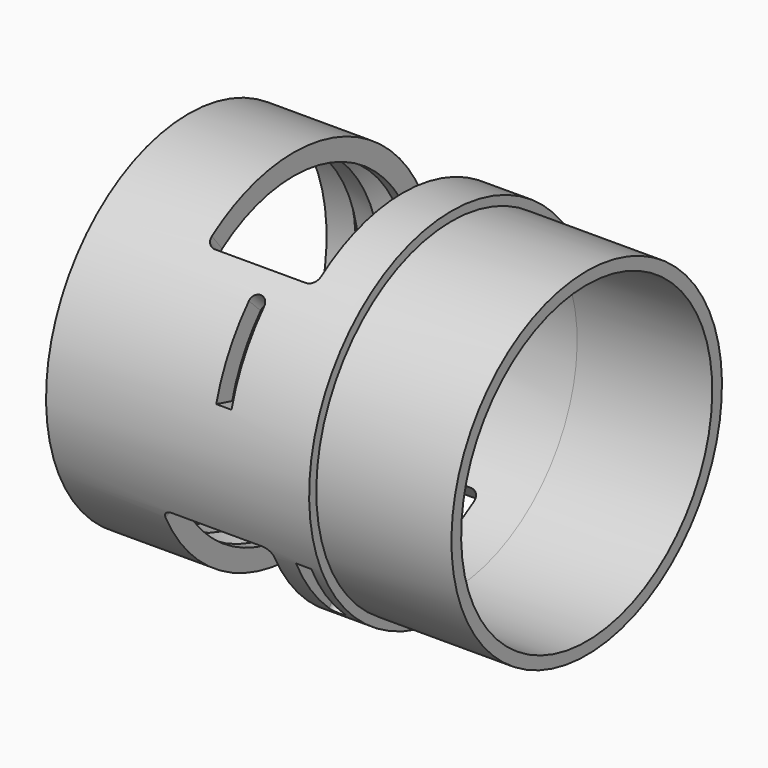
from build123d import *

# Parameters (mm, degrees)
F3_DEPTH  = 36.957
F4_R      = 6.35
F7_DEPTH  = 5.1562
F8_R      = 5.15619
F11_DEPTH = 5.1562
F12_R     = 5.15619


# Not quite as in the source:
# - a fillet or chamfer is up to 0.001 mm smaller than in the source, because OpenCascade refuses the exact size


with BuildPart() as f1:
    # F0 (on Front) → F1 (revolve)
    with BuildSketch(Plane.XZ):
        Polygon((-88.2352406061, 116.84), (-77.6180406061, 106.2228), (-63.2924406061, 106.2228), (-52.6752406061, 116.84), (-43.7044062913, 116.84), (-43.7044062913, 106.5403), (70.0067593939, 106.5403), (70.0067593939, 106.2228), (161.4467593939, 106.2228), (161.4467593939, 114.4397), (70.0067593939, 114.4397), (70.0067593939, 120.523), (-108.0472406061, 120.523), (-108.0472406061, 116.84), align=None)
    revolve(axis=Axis((26.6997593939, 0, 0), (1, 0, 0)))

    # F2 (on Right) → F3 (cut, symmetric)
    with BuildSketch(Plane.YZ):
        with BuildLine():
            Line((-79.5165483207, 101.776540644), (-60.0681501855, 76.8837261913))
            ThreePointArc((-60.0681501855, 76.8837261913), (24.428788043, 94.4591146185), (89.8107580216, 38.1224050048))
            Line((89.8107580216, 38.1224050048), (118.8889862246, 50.465380577))
            ThreePointArc((118.8889862246, 50.465380577), (32.3381508976, 125.0423515407), (-79.5165483207, 101.776540644))
        make_face()
        with BuildLine():
            ThreePointArc((60.0681501855, -76.8837261913), (-24.428788043, -94.4591146185), (-89.8107580216, -38.1224050048))
            Line((-89.8107580216, -38.1224050048), (-118.8889862246, -50.465380577))
            ThreePointArc((-118.8889862246, -50.465380577), (-32.3381508976, -125.0423515407), (79.5165483207, -101.776540644))
            Line((79.5165483207, -101.776540644), (60.0681501855, -76.8837261913))
        make_face()
    extrude(amount=F3_DEPTH, both=True, mode=Mode.SUBTRACT)

    # F4
    f4_edges = [f1.edges().sort_by_distance(p)[0] for p in [
        (36.957, -69.897063, 89.464161),
        (-36.957, -69.897063, 89.464161),
        (-36.957, 104.506435, 44.36035),
        (36.957, 104.506435, 44.36035),
        (36.957, -104.506435, -44.36035),
        (36.957, 69.897063, -89.464161),
        (-36.957, -104.506435, -44.36035),
        (-36.957, 69.897063, -89.464161),
    ]]
    fillet(f4_edges, radius=F4_R)

    # F6 (on offset) → F7 (cut, symmetric)
    with BuildSketch(Plane.YZ.offset(9.017)):
        with BuildLine():
            ThreePointArc((93.8788780653, -25.1547695639), (84.169499428, -48.5952831523), (68.7241085014, -68.7241085014))
            Line((68.7241085014, -68.7241085014), (90.3596269568, -90.3596269568))
            ThreePointArc((90.3596269568, -90.3596269568), (110.6674896962, -63.8939049666), (123.4335458995, -33.0739189427))
            Line((123.4335458995, -33.0739189427), (93.8788780653, -25.1547695639))
        make_face()
        with BuildLine():
            ThreePointArc((-92.7935106347, 24.8639462374), (-83.1963856114, 48.0334556284), (-67.9295643973, 67.9295643973))
            Line((-67.9295643973, 67.9295643973), (-89.4286909818, 89.4286909818))
            ThreePointArc((-89.4286909818, 89.4286909818), (-109.5273306353, 63.2356338259), (-122.1618637084, 32.7331727265))
            Line((-122.1618637084, 32.7331727265), (-92.7935106347, 24.8639462374))
        make_face()
    extrude(amount=F7_DEPTH, both=True, mode=Mode.SUBTRACT)

    # F8 (radius 5.1562 in the source; OpenCascade refuses exactly that, so slightly less here)
    f8_edges = [f1.edges().sort_by_distance(p)[0] for p in [
        (14.1732, 80.279, -80.279),
        (3.8608, 80.279, -80.279),
        (3.8608, -80.279, 80.279),
        (14.1732, -80.279, 80.279),
    ]]
    fillet(f8_edges, radius=F8_R)

    # F10 (on offset) → F11 (cut, symmetric)
    with BuildSketch(Plane.YZ.offset(57.277)):
        with BuildLine():
            ThreePointArc((64.781849813, 77.2040022495), (80.3789780557, 60.7977459719), (91.9209264172, 41.3241976951))
            Line((91.9209264172, 41.3241976951), (115.0678452351, 52.1177832026))
            ThreePointArc((115.0678452351, 52.1177832026), (100.6398977696, 76.3445041239), (81.1972614412, 96.7671280314))
            Line((81.1972614412, 96.7671280314), (64.781849813, 77.2040022495))
        make_face()
        with BuildLine():
            ThreePointArc((-62.1507050275, -74.0683259988), (-76.7088050422, -58.8607363245), (-87.6302951199, -40.8626777008))
            Line((-87.6302951199, -40.8626777008), (-116.6783232789, -54.4079956856))
            ThreePointArc((-116.6783232789, -54.4079956856), (-102.1365355533, -78.3721201887), (-82.7526604046, -98.6207803339))
            Line((-82.7526604046, -98.6207803339), (-62.1507050275, -74.0683259988))
        make_face()
    extrude(amount=F11_DEPTH, both=True, mode=Mode.SUBTRACT)

    # F12 (radius 5.1562 in the source; OpenCascade refuses exactly that, so slightly less here)
    f12_edges = [f1.edges().sort_by_distance(p)[0] for p in [
        (62.4332, 72.976738, 86.97029),
        (52.1208, 72.976738, 86.97029),
        (62.4332, -72.976738, -86.97029),
        (52.1208, -72.976738, -86.97029),
    ]]
    fillet(f12_edges, radius=F12_R)


solid = f1.part
